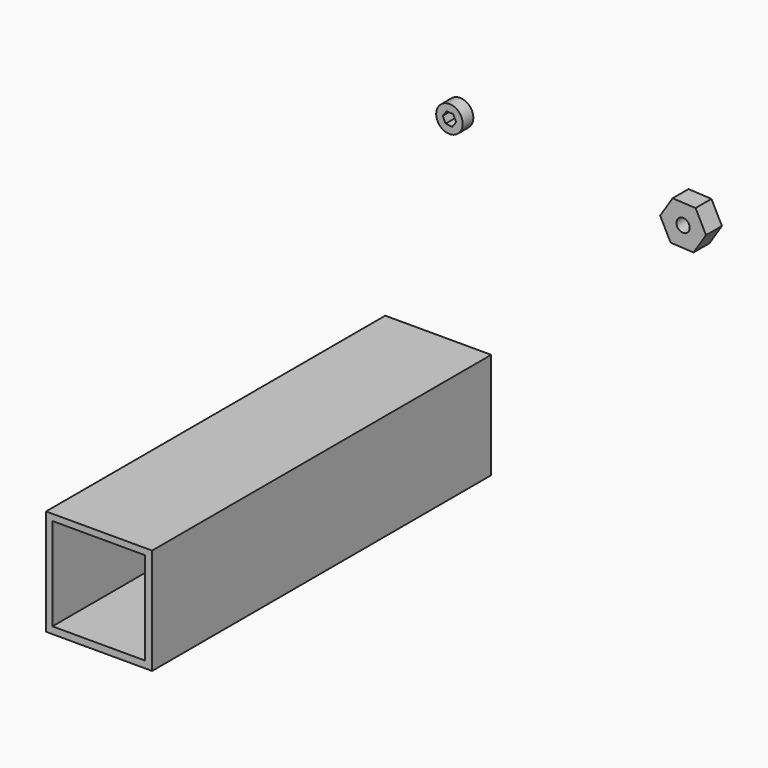
from build123d import *

# Parameters (mm, degrees)
F0_R      = 3.175
F1_DEPTH  = 3.175
F3_DEPTH  = 3.175
F6_R      = 1.5875
F7_DEPTH  = 4.7625
F8_W      = 25.4
F8_H      = 25.4
F9_DEPTH  = 101.6
F10_W     = 22.225
F10_H     = 22.225
F12_DEPTH = 101.6


# Not quite as in the source:
# - the program builds the solid bodies; features that only make, move or delete a surface that nothing else refers to are left out


with BuildPart() as f1:
    # F0 (on Front) → F1 (new body)
    with BuildSketch(Plane.XZ):
        with Locations((-30.2948281169, 38.8350300491)):
            Circle(F0_R)
    extrude(amount=F1_DEPTH)

    # F2 (on face) → F3 (cut)
    with BuildSketch(Plane.XZ.offset(3.175)):
        Polygon((-30.9442792982, 40.2931563394), (-31.8823281169, 39.0016519727), (-31.2328769355, 37.5435256824), (-29.6453769355, 37.3769037588), (-28.7073281169, 38.6684081255), (-29.3567792982, 40.1265344158), align=None)
    extrude(amount=-F3_DEPTH, mode=Mode.SUBTRACT)


with BuildPart() as f7:
    # F6 (on Front) → F7 (new body)
    with BuildSketch(Plane.XZ):
        Polygon((29.470242978, 30.7541721055), (32.4591536764, 35.3785237092), (29.9488030608, 40.2791721055), (24.4495417467, 40.5554688981), (21.4606310483, 35.9311172944), (23.9709816639, 31.0304688981), align=None)
        with Locations((26.9598923624, 35.6548205018)):
            Circle(F6_R, mode=Mode.SUBTRACT)
    extrude(amount=F7_DEPTH)


with BuildPart() as f9:
    # F8 (on Front) → F9 (new body)
    with BuildSketch(Plane.XZ):
        with Locations((-34.0042514727, -24.0096593054)):
            Rectangle(F8_W, F8_H)
    extrude(amount=F9_DEPTH)


with BuildPart() as f9_1:
    # F11: moved
    add(f9.part.moved(Location((-1.524, 0, 1.524))))

    # F10 (on face) → F12 (cut)
    with BuildSketch(Plane.XZ.offset(101.6)):
        with Locations((-35.5917514727, -22.4221593054)):
            Rectangle(F10_W, F10_H)
    extrude(amount=-F12_DEPTH, mode=Mode.SUBTRACT)


solid = Compound([f1.part, f7.part, f9_1.part])
